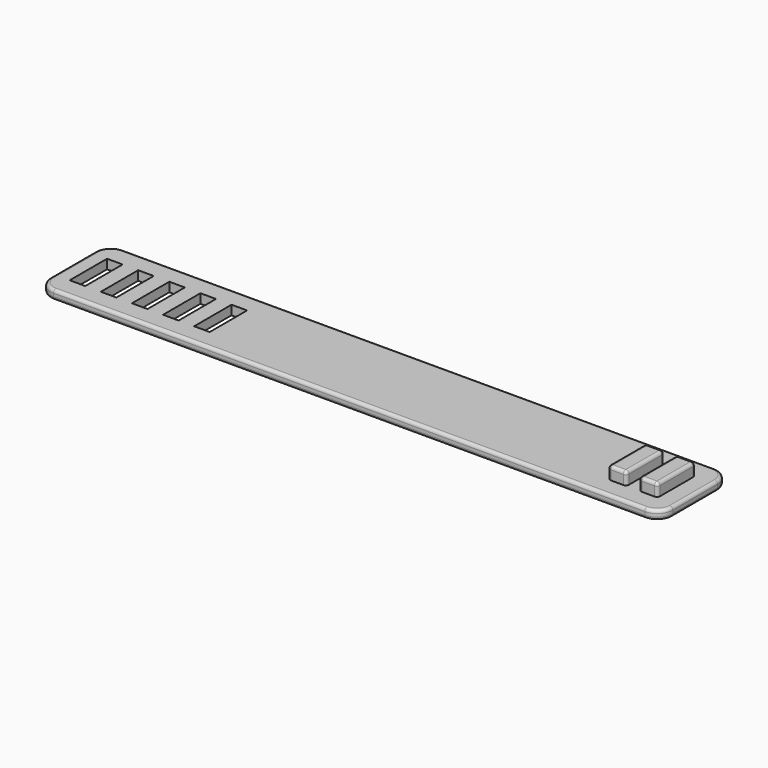
from build123d import *

# Parameters (mm, degrees)
F0_W     = 6.35
F0_H     = 19.05
F0_R     = 17.5576306553
F1_DEPTH = 3.81
F2_R     = 1.27
F3_W     = 7.62
F3_H     = 19.304
F4_DEPTH = 5.08
F5_R     = 1.27


# Not quite as in the source:
# - a feature names something its author has since deleted; it is built from what else it names


with BuildPart() as f1:
    # F0 (on Top) → F1 (new body)
    with BuildSketch(Plane.XY):
        with BuildLine():
            ThreePointArc((127, 11.43), (125.1401280605, 15.9201280605), (120.65, 17.78))
            Line((120.65, 17.78), (-120.65, 17.78))
            ThreePointArc((-120.65, 17.78), (-125.1401280605, 15.9201280605), (-127, 11.43))
            Line((-127, 11.43), (-127, -11.43))
            ThreePointArc((-127, -11.43), (-125.1401280605, -15.9201280605), (-120.65, -17.78))
            Line((-120.65, -17.78), (120.65, -17.78))
            ThreePointArc((120.65, -17.78), (125.1401280605, -15.9201280605), (127, -11.43))
            Line((127, -11.43), (127, 11.43))
        make_face()
        with Locations((-117.475, 0)):
            Rectangle(F0_W, F0_H, mode=Mode.SUBTRACT)
        with Locations((-104.775, 0)):
            Rectangle(F0_W, F0_H, mode=Mode.SUBTRACT)
        with Locations((-92.075, 0)):
            Rectangle(F0_W, F0_H, mode=Mode.SUBTRACT)
        with Locations((-79.375, 0)):
            Rectangle(F0_W, F0_H, mode=Mode.SUBTRACT)
        with Locations((-66.675, 0)):
            Rectangle(F0_W, F0_H, mode=Mode.SUBTRACT)
        with Locations((4.1378471069, 0)):
            Circle(F0_R, mode=Mode.SUBTRACT)
        with Locations((4.1378471069, 0)):
            Circle(F0_R)
    extrude(amount=F1_DEPTH)

    # F2
    f2_edges = [f1.edges().sort_by_distance(p)[0] for p in [
        (0, -17.78, 0),
        (0, -17.78, 3.81),
    ]]
    fillet(f2_edges, radius=F2_R)

    # F3 (on face) → F4 (join)
    with BuildSketch(Plane.XY.offset(3.81)):
        with Locations((102.87, 0)):
            Rectangle(F3_W, F3_H)
        with Locations((115.57, 0)):
            Rectangle(F3_W, F3_H)
    extrude(amount=F4_DEPTH)

    # F5
    f5_edges = [f1.edges().sort_by_distance(p)[0] for p in [
        (106.68, 0, 8.89),
        (102.87, -9.652, 8.89),
        (99.06, 0, 8.89),
        (102.87, 9.652, 8.89),
        (111.76, 0, 8.89),
        (119.38, 0, 8.89),
        (115.57, -9.652, 8.89),
        (115.57, 9.652, 8.89),
        (119.38, -9.652, 6.35),
        (111.76, -9.652, 6.35),
        (106.68, -9.652, 6.35),
        (99.06, -9.652, 6.35),
        (106.68, 9.652, 6.35),
        (119.38, 9.652, 6.35),
        (111.76, 9.652, 6.35),
        (99.06, 9.652, 6.35),
    ]]
    fillet(f5_edges, radius=F5_R)


solid = f1.part
